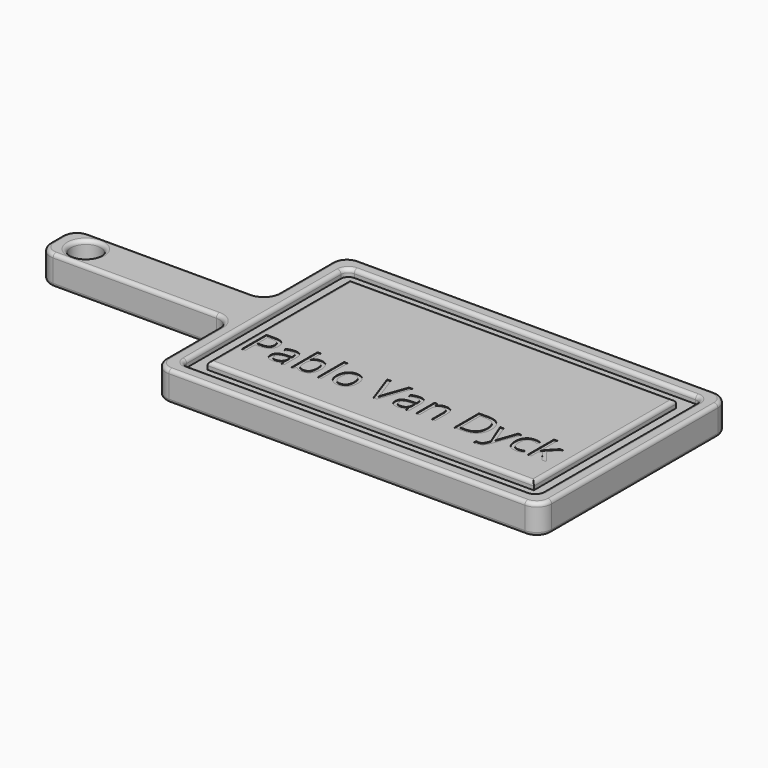
from build123d import *

# Parameters (mm, degrees)
F0_W         = 165.1
F0_H         = 38.1
F1_DEPTH     = 25.4
F2_R         = 12.7
F3_DEPTH     = 25.4
F4_W         = 279.4
F4_H         = 12.7
F4_W_2       = 12.7
F5_DEPTH     = 6.35
F6_R         = 6.35
F7_R         = 12.7
F8_R         = 3.17499
F9_TEXT_SIZE = 37.0376478247
F10_DEPTH    = 0.508


# Not quite as in the source:
# - a fillet or chamfer is up to 0.001 mm smaller than in the source, because OpenCascade refuses the exact size
# - Text() gives the source's letters only with a copy of the font that has no kerning and outlines rounded to 1/6400 em; it was checked with that copy


with BuildPart() as f1:
    # F0 (on Top) → F1 (new body)
    with BuildSketch(Plane.XY):
        Polygon((0, 82.55), (0, 0), (330.2, 0), (330.2, 203.2), (0, 203.2), (0, 120.65), align=None)
        with Locations((-82.55, 101.6)):
            Rectangle(F0_W, F0_H)
    extrude(amount=F1_DEPTH)

    # F2 (on face) → F3 (cut)
    with BuildSketch(Plane.XY.offset(25.4)):
        with Locations((-139.7, 101.6)):
            Circle(F2_R)
    extrude(amount=-F3_DEPTH, mode=Mode.SUBTRACT)

    # F4 (on face) → F5 (cut)
    with BuildSketch(Plane.XY.offset(25.4)):
        Polygon((25.4, 177.8), (12.7, 177.8), (12.7, 12.7), (317.5, 12.7), (317.5, 177.8), (304.8, 177.8), (304.8, 25.4), (25.4, 25.4), align=None)
        with Locations((165.1, 184.15)):
            Rectangle(F4_W, F4_H)
        with Locations((311.15, 184.15)):
            Rectangle(F4_W_2, F4_H)
        with Locations((19.05, 184.15)):
            Rectangle(F4_W_2, F4_H)
    extrude(amount=-F5_DEPTH, mode=Mode.SUBTRACT)

    # F6
    f6_edges = [f1.edges().sort_by_distance(p)[0] for p in [
        (12.7, 190.5, 22.225),
        (317.5, 190.5, 22.225),
        (12.7, 12.7, 22.225),
        (317.5, 12.7, 22.225),
    ]]
    fillet(f6_edges, radius=F6_R)

    # F7
    f7_edges = [f1.edges().sort_by_distance(p)[0] for p in [
        (-165.1, 82.55, 12.7),
        (0, 0, 12.7),
        (-165.1, 120.65, 12.7),
        (0, 203.2, 12.7),
        (330.2, 0, 12.7),
        (330.2, 203.2, 12.7),
        (0, 120.65, 12.7),
        (0, 82.55, 12.7),
    ]]
    fillet(f7_edges, radius=F7_R)

    # F8 (radius 3.175 in the source; OpenCascade refuses exactly that, so slightly less here)
    f8_edges = [f1.edges().sort_by_distance(p)[0] for p in [
        (25.4, 101.6, 25.4),
        (165.1, 177.8, 25.4),
        (304.8, 101.6, 25.4),
        (165.1, 25.4, 25.4),
        (0, 41.275, 25.4),
        (-3.719744, 78.830256, 25.4),
        (3.719744, 3.719744, 25.4),
        (-82.55, 82.55, 25.4),
        (165.1, 0, 25.4),
        (-161.380256, 86.269744, 25.4),
        (326.480256, 3.719744, 25.4),
        (-165.1, 101.6, 25.4),
        (330.2, 101.6, 25.4),
        (-161.380256, 116.930256, 25.4),
        (326.480256, 199.480256, 25.4),
        (-82.55, 120.65, 25.4),
        (165.1, 203.2, 25.4),
        (-3.719744, 124.369744, 25.4),
        (3.719744, 199.480256, 25.4),
        (0, 161.925, 25.4),
        (165.1, 190.5, 25.4),
        (315.640128, 188.640128, 25.4),
        (14.559872, 188.640128, 25.4),
        (317.5, 101.6, 25.4),
        (12.7, 101.6, 25.4),
        (315.640128, 14.559872, 25.4),
        (14.559872, 14.559872, 25.4),
        (165.1, 12.7, 25.4),
        (-152.4, 101.6, 25.4),
        (0, 41.275, 0),
        (-3.719744, 78.830256, 0),
        (3.719744, 3.719744, 0),
        (-82.55, 82.55, 0),
        (165.1, 0, 0),
        (-161.380256, 86.269744, 0),
        (326.480256, 3.719744, 0),
        (-165.1, 101.6, 0),
        (330.2, 101.6, 0),
        (-161.380256, 116.930256, 0),
        (326.480256, 199.480256, 0),
        (-82.55, 120.65, 0),
        (165.1, 203.2, 0),
        (-3.719744, 124.369744, 0),
        (3.719744, 199.480256, 0),
        (0, 161.925, 0),
        (-152.4, 101.6, 0),
    ]]
    fillet(f8_edges, radius=F8_R)

    # F9 (on face) → F10 (cut)
    with BuildSketch(Plane.XY.offset(25.4)):
        with Locations((28.575, 53.5622579018)):
            Text('Pablo Van Dyck', F9_TEXT_SIZE, font='Open Sans', text_align=(TextAlign.LEFT, TextAlign.BOTTOM))
    extrude(amount=-F10_DEPTH, mode=Mode.SUBTRACT)


solid = f1.part
